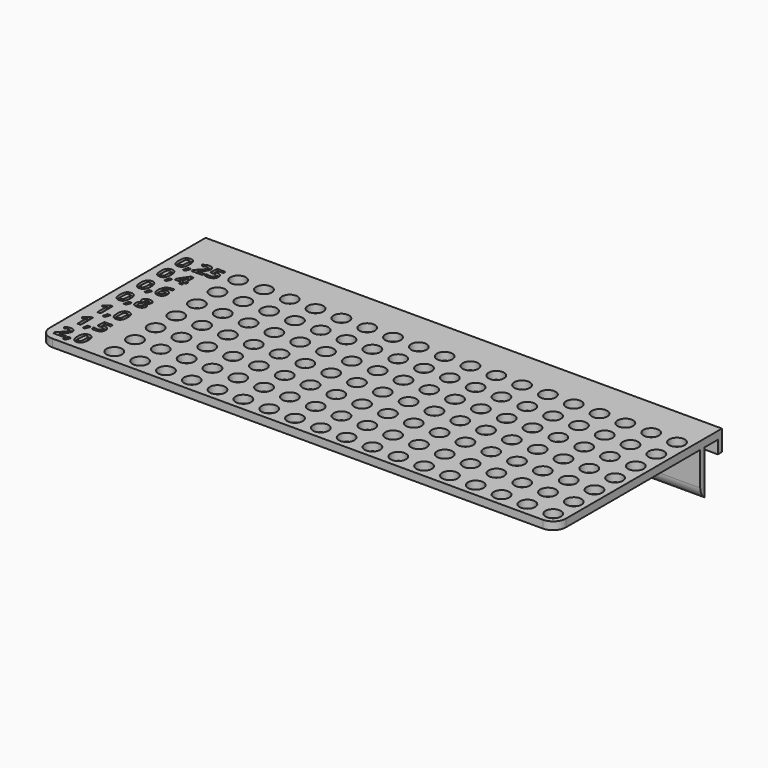
from build123d import *

# Parameters (mm, degrees)
F0_W           = 200
F0_H           = 70
F1_DEPTH       = 3
F3_D           = 6
F4_D           = 6
F5_TEXT_SIZE   = 8.3924995528
F5_TEXT_SIZE_2 = 8.1527098599
F5_TEXT_SIZE_3 = 8.2422905209
F5_TEXT_SIZE_4 = 8.2590306085
F5_TEXT_SIZE_5 = 8.2643310881
F5_TEXT_SIZE_6 = 8.3168171521
F6_DEPTH       = 1
F7_W           = 200
F7_H           = 20
F8_DEPTH       = 2
F9_W           = 200
F9_H           = 3
F10_DEPTH      = 6.5
F11_W          = 200
F11_H          = 8
F12_DEPTH      = 2
F13_T1_DEPTH   = 28
F13_T3_DEPTH   = 220


# Not quite as in the source:
# - a fillet or chamfer that OpenCascade refuses, or shapes differently, is made with other operations: its cross-section is extruded or revolved along the edge and cut away or added
# - Text() gives the source's letters only with a copy of the font that has no kerning and outlines rounded to 1/6400 em; it was checked with that copy


with BuildPart() as f1:
    # F0 (on Top) → F1 (new body)
    with BuildSketch(Plane.XY):
        with Locations((-4.0647253394, 40.1793128252)):
            Rectangle(F0_W, F0_H)
    extrude(amount=F1_DEPTH)

    # F3 (through all)
    with Locations(Plane.XY.offset(3)):
        with Locations((-39.0647253394, 70.1793128252), (-49.0647253394, 10.2224021936), (-69.0647253394, 50.2224021936), (-69.0647253394, 60.1793128252), (0.9352746606, 50.2224021936), (-79.0647253394, 50.2224021936), (-79.0647253394, 30.2224021936), (-79.0647253394, 40.2224021936), (-9.0647253394, 10.2224021936), (-69.0647253394, 10.2224021936), (-69.0647253394, 20.2224021936), (-59.0647253394, 50.2224021936), (-29.0647253394, 10.2224021936), (-79.0647253394, 60.1793128252), (10.9352746606, 70.1793128252), (-19.0647253394, 30.2224021936), (-59.0647253394, 70.1793128252), (-69.0647253394, 70.1793128252), (-19.0647253394, 40.2224021936), (-19.0647253394, 20.2224021936), (10.9352746606, 10.2224021936), (-69.0647253394, 30.2224021936), (-69.0647253394, 40.2224021936), (-59.0647253394, 40.2224021936), (-79.0647253394, 70.1793128252), (10.9352746606, 20.2224021936), (-29.0647253394, 70.1793128252), (0.9352746606, 70.1793128252), (-9.0647253394, 20.2224021936), (-9.0647253394, 40.2224021936), (10.9352746606, 60.1793128252), (10.9352746606, 40.2224021936), (-49.0647253394, 20.2224021936), (-49.0647253394, 60.1793128252), (-19.0647253394, 60.1793128252), (-19.0647253394, 70.1793128252), (-9.0647253394, 60.1793128252), (10.9352746606, 30.2224021936), (-29.0647253394, 40.2224021936), (-59.0647253394, 30.2224021936), (-39.0647253394, 40.2224021936), (-39.0647253394, 10.2224021936), (-49.0647253394, 40.2224021936), (-49.0647253394, 50.2224021936), (0.9352746606, 60.1793128252), (-59.0647253394, 10.2224021936), (-49.0647253394, 30.2224021936), (0.9352746606, 20.2224021936), (-79.0647253394, 20.2224021936), (-9.0647253394, 30.2224021936), (-29.0647253394, 60.1793128252), (0.9352746606, 40.2224021936), (-39.0647253394, 60.1793128252), (-39.0647253394, 20.2224021936), (-49.0647253394, 70.1793128252), (-39.0647253394, 50.2224021936), (-29.0647253394, 50.2224021936), (0.9352746606, 30.2224021936), (10.9352746606, 50.2224021936), (-19.0647253394, 10.2224021936), (-29.0647253394, 30.2224021936), (-9.0647253394, 70.1793128252), (-9.0647253394, 50.2224021936), (-19.0647253394, 50.2224021936), (-39.0647253394, 30.2224021936), (-29.0647253394, 20.2224021936), (0.9352746606, 10.2224021936), (-79.0647253394, 10.2224021936), (-59.0647253394, 20.2224021936), (-59.0647253394, 60.1793128252), (20.9352746606, 70.1793128252), (30.9352746606, 70.1793128252), (20.9352746606, 50.2224021936), (20.9352746606, 40.2224021936), (30.9352746606, 50.2224021936), (30.9352746606, 20.2224021936), (20.9352746606, 30.2224021936), (30.9352746606, 40.2224021936), (20.9352746606, 10.2224021936), (30.9352746606, 10.2224021936), (30.9352746606, 60.1793128252), (20.9352746606, 60.1793128252), (30.9352746606, 30.2224021936), (20.9352746606, 20.2224021936), (40.9352746606, 20.2224021936), (40.9352746606, 10.2224021936), (50.9352746606, 10.2224021936), (50.9352746606, 20.2224021936)):
            Hole(F3_D / 2)

    # F4 (through all)
    with Locations(Plane.XY.offset(3)):
        with Locations((50.9352746606, 70.1793128252), (40.9352746606, 70.1793128252), (50.9352746606, 50.2224021936), (40.9352746606, 50.2224021936), (50.9352746606, 40.2224021936), (40.9352746606, 60.1793128252), (40.9352746606, 30.2224021936), (40.9352746606, 40.2224021936), (50.9352746606, 60.1793128252), (50.9352746606, 30.2224021936), (70.9352746606, 20.2224021936), (60.9352746606, 50.2224021936), (60.9352746606, 60.1793128252), (60.9352746606, 10.2224021936), (70.9352746606, 60.1793128252), (60.9352746606, 40.2224021936), (70.9352746606, 50.2224021936), (70.9352746606, 30.2224021936), (70.9352746606, 10.2224021936), (70.9352746606, 70.1793128252), (60.9352746606, 70.1793128252), (60.9352746606, 30.2224021936), (60.9352746606, 20.2224021936), (70.9352746606, 40.2224021936), (90.9352746606, 40.2224021936), (80.9352746606, 10.2224021936), (90.9352746606, 50.2224021936), (80.9352746606, 70.1793128252), (90.9352746606, 20.2224021936), (90.9352746606, 70.1793128252), (80.9352746606, 60.1793128252), (80.9352746606, 30.2224021936), (80.9352746606, 40.2224021936), (80.9352746606, 50.2224021936), (90.9352746606, 30.2224021936), (80.9352746606, 20.2224021936), (90.9352746606, 10.2224021936), (90.9352746606, 60.1793128252)):
            Hole(F4_D / 2)

    # F5 (on face) → F6 (cut)
    with BuildSketch(Plane.XY.offset(3)):
        with Locations((-101.3949885964, 66.03500247)):
            Text('0,25', F5_TEXT_SIZE, font='Open Sans', font_style=FontStyle.BOLD, text_align=(TextAlign.LEFT, TextAlign.BOTTOM))
        with Locations((-101.3949885964, 57.2300814092)):
            Text('0,4', F5_TEXT_SIZE_2, font='Open Sans', font_style=FontStyle.BOLD, text_align=(TextAlign.LEFT, TextAlign.BOTTOM))
        with Locations((-101.3949885964, 47.4253327022)):
            Text('0,6', F5_TEXT_SIZE_3, font='Open Sans', font_style=FontStyle.BOLD, text_align=(TextAlign.LEFT, TextAlign.BOTTOM))
        with Locations((-101.3949885964, 37.5229654384)):
            Text('0,8', F5_TEXT_SIZE_4, font='Open Sans', font_style=FontStyle.BOLD, text_align=(TextAlign.LEFT, TextAlign.BOTTOM))
        with Locations((-101.3949885964, 27.2205069306)):
            Text('1,0', F5_TEXT_SIZE_5, font='Open Sans', font_style=FontStyle.BOLD, text_align=(TextAlign.LEFT, TextAlign.BOTTOM))
        with Locations((-101.3949885964, 17.539756875)):
            Text('1,5', F5_TEXT_SIZE_6, font='Open Sans', font_style=FontStyle.BOLD, text_align=(TextAlign.LEFT, TextAlign.BOTTOM))
        with Locations((-101.3949885964, 8.1143935787)):
            Text('2,0', F5_TEXT_SIZE_5, font='Open Sans', font_style=FontStyle.BOLD, text_align=(TextAlign.LEFT, TextAlign.BOTTOM))
    extrude(amount=-F6_DEPTH, mode=Mode.SUBTRACT)

    # F7 (on face) → F8 (join)
    with BuildSketch(Plane(origin=(0, 75.1793128252, 0), x_dir=(-1, 0, 0), z_dir=(0, 1, 0))):
        with Locations((4.0647253394, -7)):
            Rectangle(F7_W, F7_H)
    extrude(amount=F8_DEPTH)

    # F9 (on face) → F10 (join)
    with BuildSketch(Plane(origin=(0, 77.1793128252, 0), x_dir=(-1, 0, 0), z_dir=(0, 1, 0))):
        with Locations((4.0647253394, 1.5)):
            Rectangle(F9_W, F9_H)
    extrude(amount=F10_DEPTH)

    # F11 (on face) → F12 (join)
    with BuildSketch(Plane(origin=(0, 83.6793128252, 0), x_dir=(-1, 0, 0), z_dir=(0, 1, 0))):
        with Locations((4.0647253394, -1)):
            Rectangle(F11_W, F11_H)
    extrude(amount=F12_DEPTH)

    # F13: fillet of radius 5 on 3 edges, made by hand

    # F13_s2 → F13_t1 (cut)
    with BuildSketch(Plane.XY.offset(-12.5)):
        with BuildLine():
            ThreePointArc((-99.0647253394, 5.1793128252), (-102.6002592453, 6.6437789193), (-104.0647253394, 10.1793128252))
            Line((-104.0647253394, 10.1793128252), (-104.0647253394, 5.1793128252))
            Line((-104.0647253394, 5.1793128252), (-99.0647253394, 5.1793128252))
        make_face()
        with BuildLine():
            ThreePointArc((90.9352746606, 5.1793128252), (94.4708085665, 6.6437789193), (95.9352746606, 10.1793128252))
            Line((95.9352746606, 10.1793128252), (95.9352746606, 5.1793128252))
            Line((95.9352746606, 5.1793128252), (90.9352746606, 5.1793128252))
        make_face()
    extrude(amount=F13_T1_DEPTH, mode=Mode.SUBTRACT)

    # F13_s4 → F13_t3 (cut)
    with BuildSketch(Plane.YZ.offset(-114.0647253394)):
        with BuildLine():
            ThreePointArc((77.1793128252, -17), (75.7071768702, -15.2360679775), (75.1793128252, -13))
            Line((75.1793128252, -13), (75.1793128252, -17))
            Line((75.1793128252, -17), (77.1793128252, -17))
        make_face()
    extrude(amount=F13_T3_DEPTH, mode=Mode.SUBTRACT)


solid = f1.part
